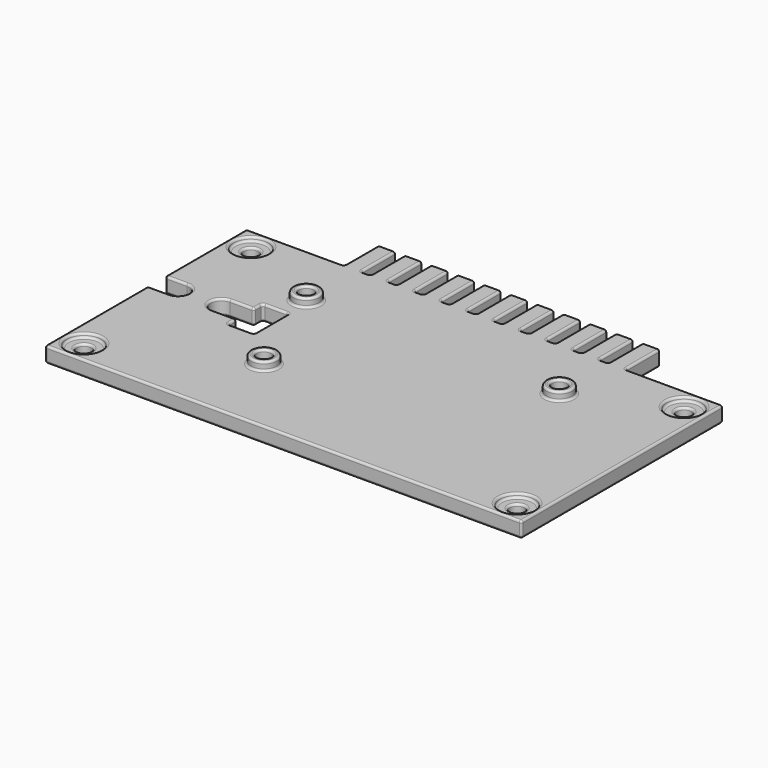
from build123d import *

# Parameters (mm, degrees)
F0_R     = 1.7
F0_W     = 4
F0_H     = 10
F1_DEPTH = 3.6
F2_R     = 4
F2_R_2   = 1.7
F3_DEPTH = 1
F2_R_3   = 3
F4_DEPTH = 2
F5_DEPTH = 25
F6_R     = 0.49999


# Not quite as in the source:
# - a fillet or chamfer is up to 0.001 mm smaller than in the source, because OpenCascade refuses the exact size
# - a feature names something its author has since deleted; it is built from what else it names


with BuildPart() as f1:
    # F0 (on Top) → F1 (new body)
    with BuildSketch(Plane.XY):
        Polygon((-31.75, -29.09), (31.75, -29.09), (55, -29.09), (55, -19.09), (55, 19.09), (55, 29.09), (32.5, 29.09), (28.5, 29.09), (26.4, 29.09), (22.4, 29.09), (20.3, 29.09), (16.3, 29.09), (14.2, 29.09), (10.2, 29.09), (8.1, 29.09), (4.1, 29.09), (2, 29.09), (-2, 29.09), (-4.1, 29.09), (-8.1, 29.09), (-10.2, 29.09), (-14.2, 29.09), (-16.3, 29.09), (-20.3, 29.09), (-22.4, 29.09), (-26.4, 29.09), (-28.5, 29.09), (-32.5, 29.09), (-55, 29.09), (-55, 19.09), (-55, -19.09), (-55, -29.09), align=None)
        with Locations((-50, -24.09)):
            Circle(F0_R, mode=Mode.SUBTRACT)
        with Locations((-19.685, -10.04)):
            Circle(F0_R, mode=Mode.SUBTRACT)
        with Locations((50, -24.09)):
            Circle(F0_R, mode=Mode.SUBTRACT)
        with Locations((-29.21, 14.09)):
            Circle(F0_R, mode=Mode.SUBTRACT)
        with Locations((-50, 24.09)):
            Circle(F0_R, mode=Mode.SUBTRACT)
        with Locations((29.21, 14.09)):
            Circle(F0_R, mode=Mode.SUBTRACT)
        with Locations((50, 24.09)):
            Circle(F0_R, mode=Mode.SUBTRACT)
        with Locations((-30.5, 34.09)):
            Rectangle(F0_W, F0_H)
        with Locations((-24.4, 34.09)):
            Rectangle(F0_W, F0_H)
        with Locations((-18.3, 34.09)):
            Rectangle(F0_W, F0_H)
        with Locations((-12.2, 34.09)):
            Rectangle(F0_W, F0_H)
        with Locations((-6.1, 34.09)):
            Rectangle(F0_W, F0_H)
        with Locations((0, 34.09)):
            Rectangle(F0_W, F0_H)
        with Locations((6.1, 34.09)):
            Rectangle(F0_W, F0_H)
        with Locations((12.2, 34.09)):
            Rectangle(F0_W, F0_H)
        with Locations((18.3, 34.09)):
            Rectangle(F0_W, F0_H)
        with Locations((24.4, 34.09)):
            Rectangle(F0_W, F0_H)
        with Locations((30.5, 34.09)):
            Rectangle(F0_W, F0_H)
    extrude(amount=F1_DEPTH)

    # F2 (on face) → F3 (cut)
    with BuildSketch(Plane.XY.offset(3.6)):
        with Locations((-50, 24.09)):
            Circle(F2_R)
        with Locations((-50, 24.09)):
            Circle(F2_R_2, mode=Mode.SUBTRACT)
        with Locations((50, 24.09)):
            Circle(F2_R)
        with Locations((50, 24.09)):
            Circle(F2_R_2, mode=Mode.SUBTRACT)
        with Locations((50, -24.09)):
            Circle(F2_R)
        with Locations((50, -24.09)):
            Circle(F2_R_2, mode=Mode.SUBTRACT)
        with Locations((-50, -24.09)):
            Circle(F2_R)
        with Locations((-50, -24.09)):
            Circle(F2_R_2, mode=Mode.SUBTRACT)
    extrude(amount=-F3_DEPTH, mode=Mode.SUBTRACT)

    # F2 (on face) → F4 (join)
    with BuildSketch(Plane.XY.offset(3.6)):
        with Locations((-29.21, 14.09)):
            Circle(F2_R_3)
        with Locations((-29.21, 14.09)):
            Circle(F2_R_2, mode=Mode.SUBTRACT)
        with Locations((-19.685, -10.04)):
            Circle(F2_R_3)
        with Locations((-19.685, -10.04)):
            Circle(F2_R_2, mode=Mode.SUBTRACT)
        with Locations((29.21, 14.09)):
            Circle(F2_R_3)
        with Locations((29.21, 14.09)):
            Circle(F2_R_2, mode=Mode.SUBTRACT)
    extrude(amount=F4_DEPTH)

    # F2 (on face) → F5 (cut)
    with BuildSketch(Plane.XY.offset(3.6)):
        Polygon((-34.5, 8.09), (-34.5, 5.59), (-34.5, 0.59), (-34.5, -1.91), (-28.5, -1.91), (-28.5, 8.09), align=None)
        with BuildLine():
            ThreePointArc((-40, 5.59), (-38.232233047, 4.857766953), (-37.5, 3.09))
            ThreePointArc((-37.5, 3.09), (-38.232233047, 1.322233047), (-40, 0.59))
            Line((-40, 0.59), (-34.5, 0.59))
            Line((-34.5, 0.59), (-34.5, 5.59))
            Line((-34.5, 5.59), (-40, 5.59))
        make_face()
        with BuildLine():
            ThreePointArc((-40, 0.59), (-38.232233047, 1.322233047), (-37.5, 3.09))
            ThreePointArc((-37.5, 3.09), (-38.232233047, 4.857766953), (-40, 5.59))
            ThreePointArc((-40, 5.59), (-42.5, 3.09), (-40, 0.59))
        make_face()
        with BuildLine():
            ThreePointArc((-50, 0.59), (-48.232233047, 1.322233047), (-47.5, 3.09))
            ThreePointArc((-47.5, 3.09), (-48.232233047, 4.857766953), (-50, 5.59))
            ThreePointArc((-50, 5.59), (-52.5, 3.09), (-50, 0.59))
        make_face()
        with BuildLine():
            ThreePointArc((-50, 0.59), (-52.5, 3.09), (-50, 5.59))
            Line((-50, 5.59), (-55, 5.59))
            Line((-55, 5.59), (-55, 0.59))
            Line((-55, 0.59), (-50, 0.59))
        make_face()
    extrude(amount=-F5_DEPTH, mode=Mode.SUBTRACT)

    # F6 (radius 0.5 in the source; OpenCascade refuses exactly that, so slightly less here)
    f6_edges = [f1.edges().sort_by_distance(p)[0] for p in [
        (43.75, 29.09, 3.6),
        (-43.75, 29.09, 3.6),
        (-27.45, 29.09, 3.6),
        (-21.35, 29.09, 3.6),
        (-15.25, 29.09, 3.6),
        (-9.15, 29.09, 3.6),
        (-3.05, 29.09, 3.6),
        (3.05, 29.09, 3.6),
        (9.15, 29.09, 3.6),
        (15.25, 29.09, 3.6),
        (21.35, 29.09, 3.6),
        (27.45, 29.09, 3.6),
        (-51.7, 24.09, 0),
        (-48.3, 24.09, 1.3),
        (-51.7, 24.09, 2.6),
        (-30.91, 14.09, 0),
        (-27.51, 14.09, 2.8),
        (-30.91, 14.09, 5.6),
        (-21.385, -10.04, 0),
        (-17.985, -10.04, 2.8),
        (-21.385, -10.04, 5.6),
        (-51.7, -24.09, 0),
        (-48.3, -24.09, 1.3),
        (-51.7, -24.09, 2.6),
        (27.51, 14.09, 0),
        (30.91, 14.09, 2.8),
        (27.51, 14.09, 5.6),
        (48.3, 24.09, 0),
        (51.7, 24.09, 1.3),
        (48.3, 24.09, 2.6),
        (48.3, -24.09, 0),
        (51.7, -24.09, 1.3),
        (48.3, -24.09, 2.6),
        (55, -29.09, 1.8),
        (55, 29.09, 1.8),
        (55, 0, 0),
        (55, 0, 3.6),
        (-55, -29.09, 1.8),
        (0, -29.09, 0),
        (0, -29.09, 3.6),
        (-55, -14.25, 0),
        (-55, -14.25, 3.6),
        (-55, 0.59, 1.8),
        (43.75, 29.09, 0),
        (-43.75, 29.09, 0),
        (-27.45, 29.09, 0),
        (-21.35, 29.09, 0),
        (-15.25, 29.09, 0),
        (-9.15, 29.09, 0),
        (-3.05, 29.09, 0),
        (3.05, 29.09, 0),
        (9.15, 29.09, 0),
        (15.25, 29.09, 0),
        (21.35, 29.09, 0),
        (27.45, 29.09, 0),
        (-34.5, 6.84, 3.6),
        (-34.5, 5.59, 1.8),
        (-34.5, 6.84, 0),
        (-34.5, 8.09, 1.8),
        (-31.5, 8.09, 3.6),
        (-31.5, 8.09, 0),
        (-28.5, 8.09, 1.8),
        (-28.5, 3.09, 3.6),
        (-28.5, 3.09, 0),
        (-28.5, -1.91, 1.8),
        (-31.5, -1.91, 3.6),
        (-31.5, -1.91, 0),
        (-34.5, -1.91, 1.8),
        (-37.25, 0.59, 3.6),
        (-34.5, 0.59, 1.8),
        (-37.25, 0.59, 0),
        (-40, 0.59, 1.8),
        (-42.5, 3.09, 3.6),
        (-42.5, 3.09, 0),
        (-40, 5.59, 1.8),
        (-47.5, 3.09, 3.6),
        (-50, 5.59, 1.8),
        (-47.5, 3.09, 0),
        (-50, 0.59, 1.8),
        (-37.25, 5.59, 3.6),
        (-37.25, 5.59, 0),
        (-22.685, -10.04, 5.6),
        (-22.685, -10.04, 3.6),
        (-32.21, 14.09, 3.6),
        (-32.21, 14.09, 5.6),
        (26.21, 14.09, 5.6),
        (32.21, 14.09, 4.6),
        (26.21, 14.09, 3.6),
        (54, -24.09, 3.1),
        (46, -24.09, 3.6),
        (46, -24.09, 2.6),
        (-54, -24.09, 2.6),
        (-54, -24.09, 3.6),
        (-46, 24.09, 3.1),
        (-54, 24.09, 3.6),
        (-54, 24.09, 2.6),
        (54, 24.09, 3.1),
        (46, 24.09, 3.6),
        (46, 24.09, 2.6),
        (-52.5, 5.59, 3.6),
        (-55, 5.59, 1.8),
        (-52.5, 5.59, 0),
        (-52.5, 0.59, 3.6),
        (-52.5, 0.59, 0),
        (32.5, 39.09, 1.8),
        (28.5, 39.09, 1.8),
        (30.5, 39.09, 0),
        (30.5, 39.09, 3.6),
        (26.4, 39.09, 1.8),
        (22.4, 39.09, 1.8),
        (24.4, 39.09, 0),
        (24.4, 39.09, 3.6),
        (20.3, 39.09, 1.8),
        (16.3, 39.09, 1.8),
        (18.3, 39.09, 0),
        (18.3, 39.09, 3.6),
        (14.2, 39.09, 1.8),
        (10.2, 39.09, 1.8),
        (12.2, 39.09, 0),
        (12.2, 39.09, 3.6),
        (8.1, 39.09, 1.8),
        (4.1, 39.09, 1.8),
        (6.1, 39.09, 0),
        (6.1, 39.09, 3.6),
        (2, 39.09, 1.8),
        (-4.1, 39.09, 1.8),
        (-8.1, 39.09, 1.8),
        (-6.1, 39.09, 0),
        (-6.1, 39.09, 3.6),
        (-10.2, 39.09, 1.8),
        (-14.2, 39.09, 1.8),
        (-12.2, 39.09, 0),
        (-12.2, 39.09, 3.6),
        (-16.3, 39.09, 1.8),
        (-20.3, 39.09, 1.8),
        (-18.3, 39.09, 0),
        (-18.3, 39.09, 3.6),
        (-22.4, 39.09, 1.8),
        (-26.4, 39.09, 1.8),
        (-24.4, 39.09, 0),
        (-24.4, 39.09, 3.6),
        (-28.5, 39.09, 1.8),
        (-32.5, 39.09, 1.8),
        (-30.5, 39.09, 0),
        (-30.5, 39.09, 3.6),
        (-32.5, 29.09, 1.8),
        (-55, 29.09, 1.8),
        (-26.4, 29.09, 1.8),
        (-28.5, 29.09, 1.8),
        (-20.3, 29.09, 1.8),
        (-22.4, 29.09, 1.8),
        (28.5, 29.09, 1.8),
        (26.4, 29.09, 1.8),
        (22.4, 29.09, 1.8),
        (20.3, 29.09, 1.8),
        (16.3, 29.09, 1.8),
        (14.2, 29.09, 1.8),
        (10.2, 29.09, 1.8),
        (8.1, 29.09, 1.8),
        (4.1, 29.09, 1.8),
        (2, 29.09, 1.8),
        (-2, 29.09, 1.8),
        (-4.1, 29.09, 1.8),
        (-8.1, 29.09, 1.8),
        (-10.2, 29.09, 1.8),
        (-14.2, 29.09, 1.8),
        (-16.3, 29.09, 1.8),
        (-2, 39.09, 1.8),
        (0, 39.09, 0),
        (0, 39.09, 3.6),
        (28.5, 34.09, 0),
        (28.5, 34.09, 3.6),
        (22.4, 34.09, 0),
        (22.4, 34.09, 3.6),
        (16.3, 34.09, 0),
        (16.3, 34.09, 3.6),
        (10.2, 34.09, 0),
        (10.2, 34.09, 3.6),
        (4.1, 34.09, 0),
        (4.1, 34.09, 3.6),
        (-2, 34.09, 0),
        (-2, 34.09, 3.6),
        (-8.1, 34.09, 0),
        (-8.1, 34.09, 3.6),
        (-14.2, 34.09, 0),
        (-14.2, 34.09, 3.6),
        (-20.3, 34.09, 0),
        (-20.3, 34.09, 3.6),
        (-26.4, 34.09, 0),
        (-26.4, 34.09, 3.6),
        (32.5, 29.09, 1.8),
        (32.5, 34.09, 0),
        (32.5, 34.09, 3.6),
        (-55, 17.34, 0),
        (-32.5, 34.09, 0),
        (-28.5, 34.09, 0),
        (-22.4, 34.09, 0),
        (-16.3, 34.09, 0),
        (-10.2, 34.09, 0),
        (-4.1, 34.09, 0),
        (2, 34.09, 0),
        (8.1, 34.09, 0),
        (14.2, 34.09, 0),
        (20.3, 34.09, 0),
        (26.4, 34.09, 0),
        (-34.5, -0.66, 0),
        (-55, 17.34, 3.6),
        (-32.5, 34.09, 3.6),
        (-28.5, 34.09, 3.6),
        (-22.4, 34.09, 3.6),
        (-16.3, 34.09, 3.6),
        (-10.2, 34.09, 3.6),
        (-4.1, 34.09, 3.6),
        (2, 34.09, 3.6),
        (8.1, 34.09, 3.6),
        (14.2, 34.09, 3.6),
        (20.3, 34.09, 3.6),
        (26.4, 34.09, 3.6),
        (-34.5, -0.66, 3.6),
    ]]
    fillet(f6_edges, radius=F6_R)


solid = f1.part
